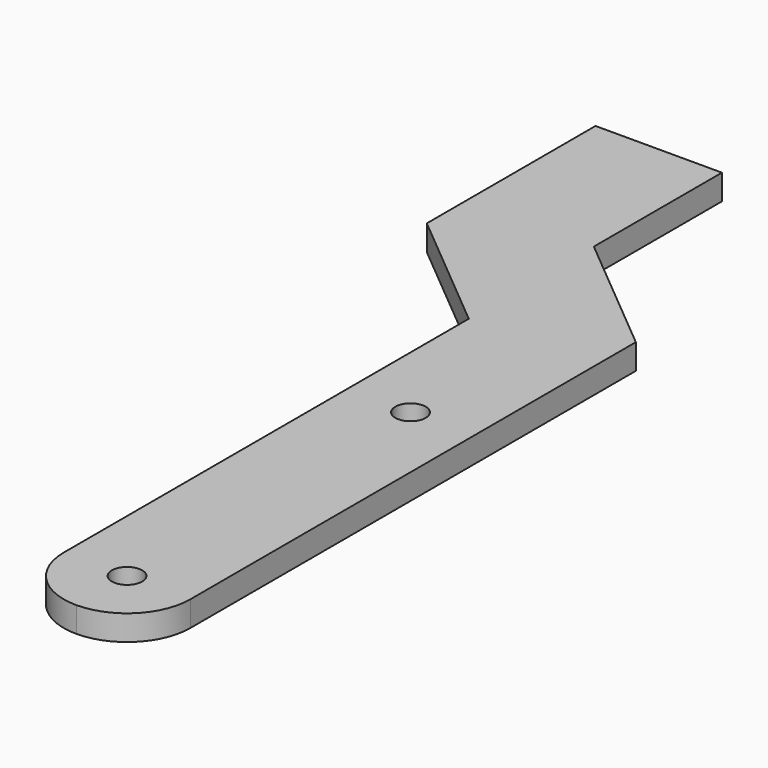
from build123d import *

# Parameters (mm, degrees)
F0_R     = 1.524
F1_DEPTH = 2.54


# Not quite as in the source:
# - a feature names something its author has since deleted; it is built from what else it names


with BuildPart() as f1:
    # F0 (on Top) → F1 (new body)
    with BuildSketch(Plane.XY):
        with BuildLine():
            Line((-19.0341994166, 42.3401940286), (-6.35, 31.75))
            Line((-6.35, 31.75), (-6.35, -19.05))
            ThreePointArc((-6.35, -19.05), (-4.4901280605, -23.5401280605), (0, -25.4))
            ThreePointArc((0, -25.4), (4.4901280605, -23.5401280605), (6.35, -19.05))
            Line((6.35, -19.05), (6.35, 36.83))
            Line((6.35, 36.83), (-6.35, 47.4333861299))
            Line((-6.35, 47.4333861299), (-6.35, 57.15))
            Line((-6.35, 57.15), (-6.35, 63.5))
            Line((-6.35, 63.5), (-19.0341994166, 63.5))
            Line((-19.0341994166, 63.5), (-19.0341994166, 42.3401940286))
        make_face()
        with Locations((0, -19.05)):
            Circle(F0_R, mode=Mode.SUBTRACT)
        with Locations((0, 16.51)):
            Circle(F0_R, mode=Mode.SUBTRACT)
    extrude(amount=F1_DEPTH)


solid = f1.part
